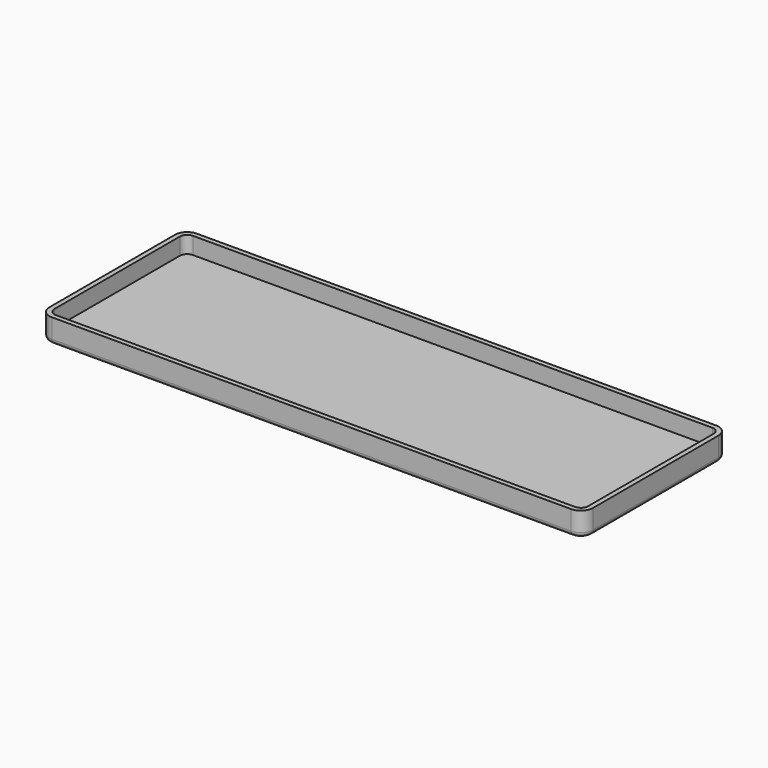
from build123d import *

# Parameters (mm, degrees)
F1_DEPTH = 3
F2_DEPTH = 10
F3_R     = 2


# Not quite as in the source:
# - a feature names something its author has since deleted; it is built from what else it names


with BuildPart() as f1:
    # F0 (on Top) → F1 (new body)
    with BuildSketch(Plane.XY):
        with BuildLine():
            ThreePointArc((-44.6118305922, 5), (-43.7331509357, 2.8786796564), (-41.6118305922, 2))
            Line((-41.6118305922, 2), (173.3881694078, 2))
            ThreePointArc((173.3881694078, 2), (175.5094897514, 2.8786796564), (176.3881694078, 5))
            Line((176.3881694078, 5), (176.3881694078, 70))
            ThreePointArc((176.3881694078, 70), (175.5094897514, 72.1213203436), (173.3881694078, 73))
            Line((173.3881694078, 73), (-41.6118305922, 73))
            ThreePointArc((-41.6118305922, 73), (-43.7331509357, 72.1213203436), (-44.6118305922, 70))
            Line((-44.6118305922, 70), (-44.6118305922, 5))
        make_face()
    extrude(amount=F1_DEPTH)

    # F0 (on Top) → F2 (join)
    with BuildSketch(Plane.XY):
        with BuildLine():
            Line((173.3881694078, 75), (-41.6118305922, 75))
            ThreePointArc((-41.6118305922, 75), (-45.1473644981, 73.5355339059), (-46.6118305922, 70))
            Line((-46.6118305922, 70), (-46.6118305922, 5))
            ThreePointArc((-46.6118305922, 5), (-45.1473644981, 1.4644660941), (-41.6118305922, 0))
            Line((-41.6118305922, 0), (173.3881694078, 0))
            ThreePointArc((173.3881694078, 0), (176.9237033138, 1.4644660941), (178.3881694078, 5))
            Line((178.3881694078, 5), (178.3881694078, 70))
            ThreePointArc((178.3881694078, 70), (176.9237033138, 73.5355339059), (173.3881694078, 75))
        make_face()
        with BuildLine():
            Line((173.3881694078, 2), (-41.6118305922, 2))
            ThreePointArc((-41.6118305922, 2), (-43.7331509357, 2.8786796564), (-44.6118305922, 5))
            Line((-44.6118305922, 5), (-44.6118305922, 70))
            ThreePointArc((-44.6118305922, 70), (-43.7331509357, 72.1213203436), (-41.6118305922, 73))
            Line((-41.6118305922, 73), (173.3881694078, 73))
            ThreePointArc((173.3881694078, 73), (175.5094897514, 72.1213203436), (176.3881694078, 70))
            Line((176.3881694078, 70), (176.3881694078, 5))
            ThreePointArc((176.3881694078, 5), (175.5094897514, 2.8786796564), (173.3881694078, 2))
        make_face(mode=Mode.SUBTRACT)
    extrude(amount=F2_DEPTH)

    # F3
    f3_edges = [f1.edges().sort_by_distance(p)[0] for p in [
        (65.888169, 75, 0),
    ]]
    fillet(f3_edges, radius=F3_R)


solid = f1.part
